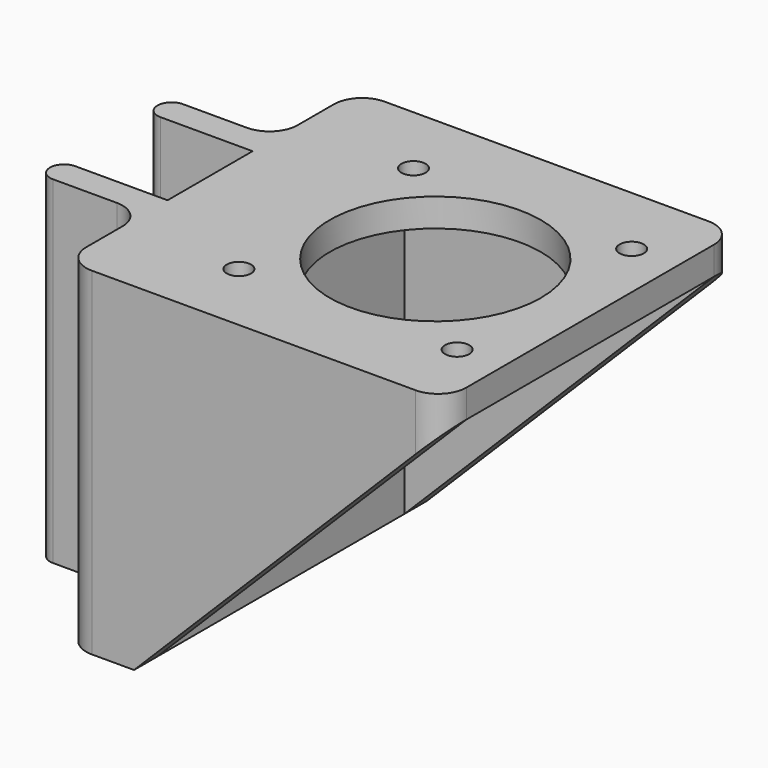
from build123d import *

# Parameters (mm, degrees)
F0_W      = 10
F0_H      = 52
F1_DEPTH  = 44
F2_W      = 54
F2_H      = 52
F3_DEPTH  = 4
F5_DEPTH  = 4
F7_DEPTH  = 4
F8_R      = 15
F8_R_2    = 1.725
F9_DEPTH  = 4
F10_R     = 1.725
F11_DEPTH = 10
F10_R_2   = 3.5
F12_DEPTH = 6
F14_W     = 15.1
F14_H     = 4
F15_DEPTH = 48
F16_R     = 1.725
F17_DEPTH = 4
F18_R     = 1.725
F19_DEPTH = 4
F20_R     = 4
F21_R     = 1.99999


# Not quite as in the source:
# - a fillet or chamfer is up to 0.001 mm smaller than in the source, because OpenCascade refuses the exact size
# - a feature of the source that left no trace in its solid (it failed there, or was rolled back) is left out
# - a feature names something its author has since deleted; it is built from what else it names


with BuildPart() as f1:
    # F0 (on Top) → F1 (new body)
    with BuildSketch(Plane.XY):
        with Locations((5, 26)):
            Rectangle(F0_W, F0_H)
    extrude(amount=F1_DEPTH)

    # F2 (on face) → F3 (join)
    with BuildSketch(Plane.XY.offset(44)):
        with Locations((27, 26)):
            Rectangle(F2_W, F2_H)
    extrude(amount=F3_DEPTH)

    # F4 (on face) → F5 (join)
    with BuildSketch(Plane.XZ):
        Polygon((10, 0), (54, 44), (10, 44), align=None)
    extrude(amount=-F5_DEPTH)

    # F6 (on face) → F7 (join)
    with BuildSketch(Plane(origin=(0, 52, 0), x_dir=(-1, 0, 0), z_dir=(0, 1, 0))):
        Polygon((-10, 44), (-54, 44), (-10, 0), align=None)
    extrude(amount=-F7_DEPTH)

    # F8 (on face) → F9 (cut, through all)
    with BuildSketch(Plane(origin=(0, 0, 44), x_dir=(1, 0, 0), z_dir=(0, 0, -1))):
        with Locations((32, -26)):
            Circle(F8_R)
        with Locations((16.5, -10.5)):
            Circle(F8_R_2)
        with Locations((47.5, -10.5)):
            Circle(F8_R_2)
        with Locations((47.5, -41.5)):
            Circle(F8_R_2)
        with Locations((16.5, -41.5)):
            Circle(F8_R_2)
    extrude(amount=-F9_DEPTH, mode=Mode.SUBTRACT)

    # F10 (on face) → F11 (cut)
    with BuildSketch(Plane.YZ.offset(10)):
        with Locations((26, 37)):
            Circle(F10_R)
        with Locations((26, 7)):
            Circle(F10_R)
    extrude(amount=-F11_DEPTH, mode=Mode.SUBTRACT)

    # F10 (on face) → F12 (cut)
    with BuildSketch(Plane.YZ.offset(10)):
        with Locations((26, 37)):
            Circle(F10_R_2)
        with Locations((26, 37)):
            Circle(F10_R, mode=Mode.SUBTRACT)
        with Locations((26, 7)):
            Circle(F10_R_2)
        with Locations((26, 7)):
            Circle(F10_R, mode=Mode.SUBTRACT)
    extrude(amount=-F12_DEPTH, mode=Mode.SUBTRACT)

    # F14 (on face) → F15 (join)
    with BuildSketch(Plane.XY.offset(48)):
        with Locations((-7.55, 35.55)):
            Rectangle(F14_W, F14_H)
        with Locations((-7.55, 16.45)):
            Rectangle(F14_W, F14_H)
    extrude(amount=-F15_DEPTH)

    # F16 (on face) → F17 (cut, through all)
    with BuildSketch(Plane.XZ.offset(-14.45)):
        with Locations((-7.55, 37)):
            Circle(F16_R)
        with Locations((-7.55, 7)):
            Circle(F16_R)
    extrude(amount=-F17_DEPTH, mode=Mode.SUBTRACT)

    # F18 (on face) → F19 (cut, through all)
    with BuildSketch(Plane(origin=(0, 37.55, 0), x_dir=(-1, 0, 0), z_dir=(0, 1, 0))):
        with Locations((7.55, 37)):
            Circle(F18_R)
        with Locations((7.55, 7)):
            Circle(F18_R)
    extrude(amount=-F19_DEPTH, mode=Mode.SUBTRACT)

    # F20
    f20_edges = [f1.edges().sort_by_distance(p)[0] for p in [
        (0, 14.45, 24),
        (0, 37.55, 24),
        (0, 52, 24),
        (54, 52, 46),
        (54, 0, 46),
        (0, 0, 24),
    ]]
    fillet(f20_edges, radius=F20_R)

    # F21 (radius 2 in the source; OpenCascade refuses exactly that, so slightly less here)
    f21_edges = [f1.edges().sort_by_distance(p)[0] for p in [
        (-15.1, 37.55, 24),
        (-15.1, 33.55, 24),
        (-15.1, 18.45, 24),
        (-15.1, 14.45, 24),
    ]]
    fillet(f21_edges, radius=F21_R)


solid = f1.part
